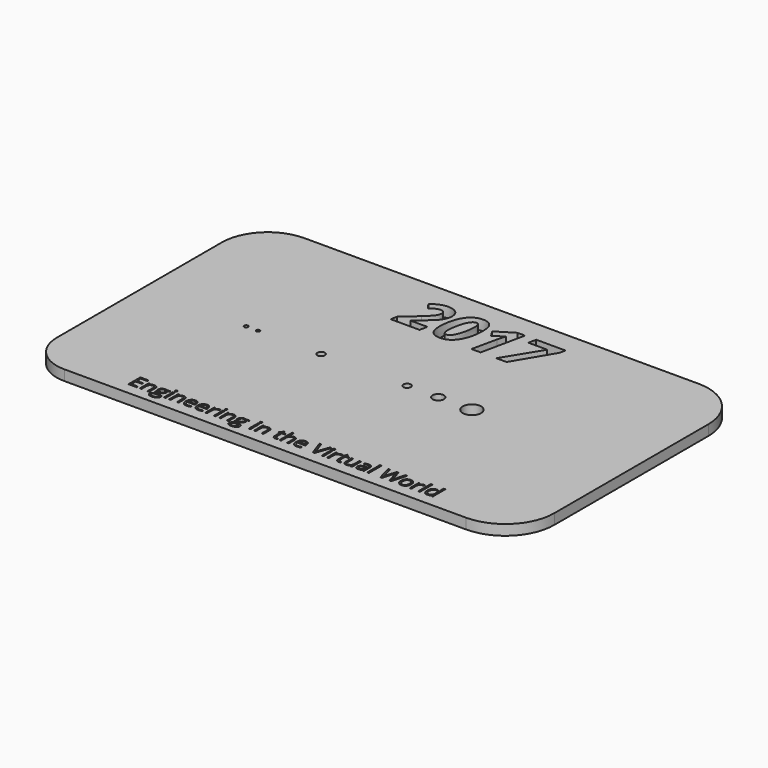
from build123d import *

# Parameters (mm, degrees)
F2_DEPTH      = 1.4
F0_R          = 0.263482103
F0_R_2        = 0.2324668937
F0_R_3        = 0.5056365473
F0_R_4        = 0.5002818197
F0_R_5        = 0.7530519003
F0_R_6        = 1.2390254218
F3_DEPTH      = 25
F3_DEPTH_BACK = 25
F4_TEXT_SIZE  = 8.3137510551
F5_DEPTH      = 25
F5_DEPTH_BACK = 25
F6_TEXT_SIZE  = 2.8120030442
F7_DEPTH      = 25
F7_DEPTH_BACK = 25


# Not quite as in the source:
# - Text() gives the source's letters only with a copy of the font that has no kerning and outlines rounded to 1/6400 em; it was checked with that copy


with BuildPart() as f2:
    # F1 (on Top) → F2 (new body)
    with BuildSketch(Plane.XY):
        with BuildLine():
            Line((-39.3541093259, -19.6518916637), (14.9259101648, -19.6518916637))
            ThreePointArc((14.9259101648, -19.6518916637), (19.6077941453, -17.7125918215), (21.5470939875, -13.030707841))
            Line((21.5470939875, -13.030707841), (21.5470939875, 12.9767265799))
            ThreePointArc((21.5470939875, 12.9767265799), (19.6161919078, 17.6383365682), (14.9545819195, 19.5692386478))
            Line((14.9545819195, 19.5692386478), (-38.2967319854, 19.5692386478))
            ThreePointArc((-38.2967319854, 19.5692386478), (-42.6724264542, 17.756766654), (-44.484898448, 13.3810721852))
            Line((-44.484898448, 13.3810721852), (-44.484898448, -14.5211025416))
            ThreePointArc((-44.484898448, -14.5211025416), (-42.982125107, -18.1491183227), (-39.3541093259, -19.6518916637))
        make_face()
    extrude(amount=F2_DEPTH)

    # F0 (on Top) → F3 (cut, two sides)
    with BuildSketch(Plane.XY) as f3_sk:
        with Locations((-30.4990187287, 0)):
            Circle(F0_R)
        with Locations((-28.8852658123, 0)):
            Circle(F0_R_2)
        with Locations((-20.3661452979, 0)):
            Circle(F0_R_3)
        with Locations((-8.7613807991, 0)):
            Circle(F0_R_4)
        with Locations((-4.5592389069, 0)):
            Circle(F0_R_5)
        Circle(F0_R_6)
    extrude(amount=-F3_DEPTH, mode=Mode.SUBTRACT)
    extrude(f3_sk.sketch, amount=F3_DEPTH_BACK, mode=Mode.SUBTRACT)

    # F4 (on face) → F5 (cut, two sides)
    with BuildSketch(Plane.XY.offset(1.4)) as f5_sk:
        with Locations((-19.4152067609, 10.7896160334)):
            Text('2017', F4_TEXT_SIZE, font='Open Sans', font_style=FontStyle.BOLDITALIC, text_align=(TextAlign.LEFT, TextAlign.BOTTOM))
    extrude(amount=-F5_DEPTH, mode=Mode.SUBTRACT)
    extrude(f5_sk.sketch, amount=F5_DEPTH_BACK, mode=Mode.SUBTRACT)

    # F6 (on face) → F7 (cut, two sides)
    with BuildSketch(Plane.XY.offset(1.4)) as f7_sk:
        with Locations((-32.213693019, -18.0835509673)):
            Text('Engineering in the Virtual World', F6_TEXT_SIZE, font='Open Sans', text_align=(TextAlign.LEFT, TextAlign.BOTTOM))
    extrude(amount=-F7_DEPTH, mode=Mode.SUBTRACT)
    extrude(f7_sk.sketch, amount=F7_DEPTH_BACK, mode=Mode.SUBTRACT)


solid = f2.part
